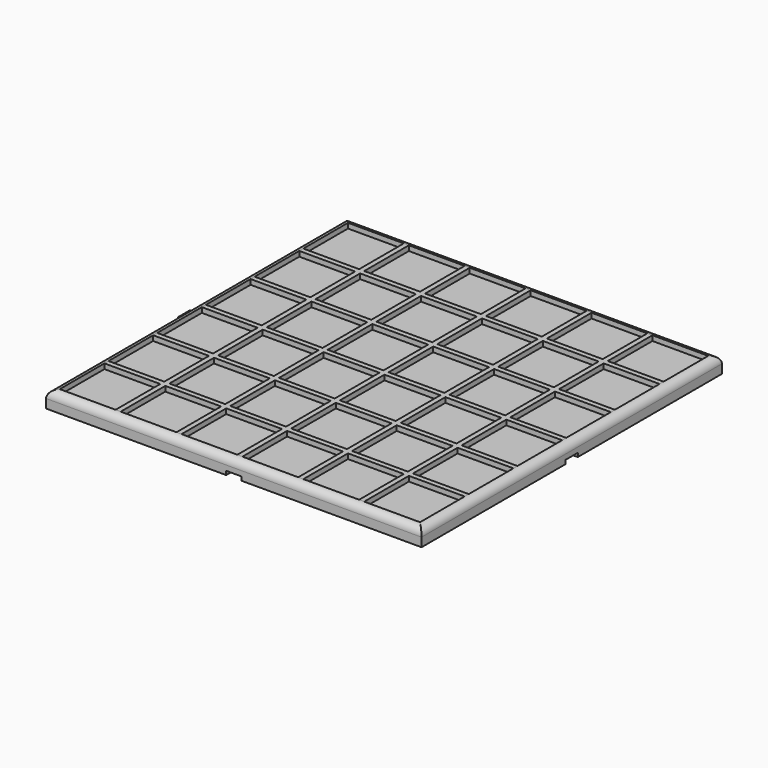
from build123d import *

# Parameters (mm, degrees)
F1_W      = 2
F1_H      = 142
F3_DEPTH  = 2
F0_W      = 148
F0_H      = 148
F0_W_2    = 142
F0_H_2    = 142
F2_W      = 142
F2_H      = 2
F5_DEPTH  = 2
F6_DEPTH  = 2
F4_W      = 148
F4_H      = 148
F7_DEPTH  = 4.5
F8_R      = 2.99999
F9_W      = 6
F9_H      = 1.5
F10_DEPTH = 5
F11_W     = 6
F11_H     = 1.5
F12_DEPTH = 5
F13_W     = 5.8
F13_H     = 1.3
F14_DEPTH = 4.8
F15_W     = 5.8
F15_H     = 1.3
F16_DEPTH = 4.8


# Not quite as in the source:
# - a fillet or chamfer is up to 0.001 mm smaller than in the source, because OpenCascade refuses the exact size


with BuildPart() as f3:
    # F1 (on Top) → F3 (new body)
    with BuildSketch(Plane.XY):
        with Locations((-48, 0)):
            Rectangle(F1_W, F1_H)
    extrude(amount=F3_DEPTH)



with BuildPart() as f3b:
    # F0 (on Top) → F3, piece 2 (new body)
    with BuildSketch(Plane.XY):
        Rectangle(F0_W, F0_H)
        Rectangle(F0_W_2, F0_H_2, mode=Mode.SUBTRACT)
    extrude(amount=F3_DEPTH)


with BuildPart() as f5:
    # F2 (on Top) → F5 (new body)
    with BuildSketch(Plane.XY):
        with Locations((0, 48)):
            Rectangle(F2_W, F2_H)
    extrude(amount=F5_DEPTH)


with BuildPart() as f5b:
    # F2 (on Top) → F5, piece 2 (new body)
    with BuildSketch(Plane.XY):
        with Locations((0, 24)):
            Rectangle(F2_W, F2_H)
    extrude(amount=F5_DEPTH)


with BuildPart() as f5c:
    # F2 (on Top) → F5, piece 3 (new body)
    with BuildSketch(Plane.XY):
        Rectangle(F2_W, F2_H)
    extrude(amount=F5_DEPTH)


with BuildPart() as f5d:
    # F2 (on Top) → F5, piece 4 (new body)
    with BuildSketch(Plane.XY):
        with Locations((0, -24)):
            Rectangle(F2_W, F2_H)
    extrude(amount=F5_DEPTH)


with BuildPart() as f5e:
    # F2 (on Top) → F5, piece 5 (new body)
    with BuildSketch(Plane.XY):
        with Locations((0, -48)):
            Rectangle(F2_W, F2_H)
    extrude(amount=F5_DEPTH)


with BuildPart() as f3_1:
    add(f3.part)

    add(f3b.part)  # F6 merges F3b

    add(f5.part)  # F6 merges F5

    add(f5b.part)  # F6 merges F5b

    add(f5c.part)  # F6 merges F5c

    add(f5d.part)  # F6 merges F5d

    add(f5e.part)  # F6 merges F5e
    # F1 (on Top) → F6 (join)
    with BuildSketch(Plane.XY):
        with Locations((-48, 0)):
            Rectangle(F1_W, F1_H)
        with Locations((-24, 0)):
            Rectangle(F1_W, F1_H)
        Rectangle(F1_W, F1_H)
        with Locations((24, 0)):
            Rectangle(F1_W, F1_H)
        with Locations((48, 0)):
            Rectangle(F1_W, F1_H)
    extrude(amount=F6_DEPTH)

    # F4 (on Top) → F7 (join)
    with BuildSketch(Plane.XY):
        Rectangle(F4_W, F4_H)
    extrude(amount=-F7_DEPTH)

    # F8 (radius 3 in the source; OpenCascade refuses exactly that, so slightly less here)
    f8_edges = [f3_1.edges().sort_by_distance(p)[0] for p in [
        (0, 74, 2),
        (-74, 0, 2),
        (0, -74, 2),
        (74, 0, 2),
    ]]
    fillet(f8_edges, radius=F8_R)

    # F9 (on face) → F10 (cut)
    with BuildSketch(Plane.YZ.offset(74)):
        with Locations((0, -3.75)):
            Rectangle(F9_W, F9_H)
    extrude(amount=-F10_DEPTH, mode=Mode.SUBTRACT)

    # F11 (on face) → F12 (cut)
    with BuildSketch(Plane.XZ.offset(74)):
        with Locations((0, -3.75)):
            Rectangle(F11_W, F11_H)
    extrude(amount=-F12_DEPTH, mode=Mode.SUBTRACT)

    # F13 (on face) → F14 (join)
    with BuildSketch(Plane(origin=(-74, 0, 0), x_dir=(0, -1, 0), z_dir=(-1, 0, 0))):
        with Locations((0, -3.85)):
            Rectangle(F13_W, F13_H)
    extrude(amount=F14_DEPTH)

    # F15 (on face) → F16 (join)
    with BuildSketch(Plane(origin=(0, 74, 0), x_dir=(-1, 0, 0), z_dir=(0, 1, 0))):
        with Locations((0, -3.85)):
            Rectangle(F15_W, F15_H)
    extrude(amount=F16_DEPTH)


solid = f3_1.part
